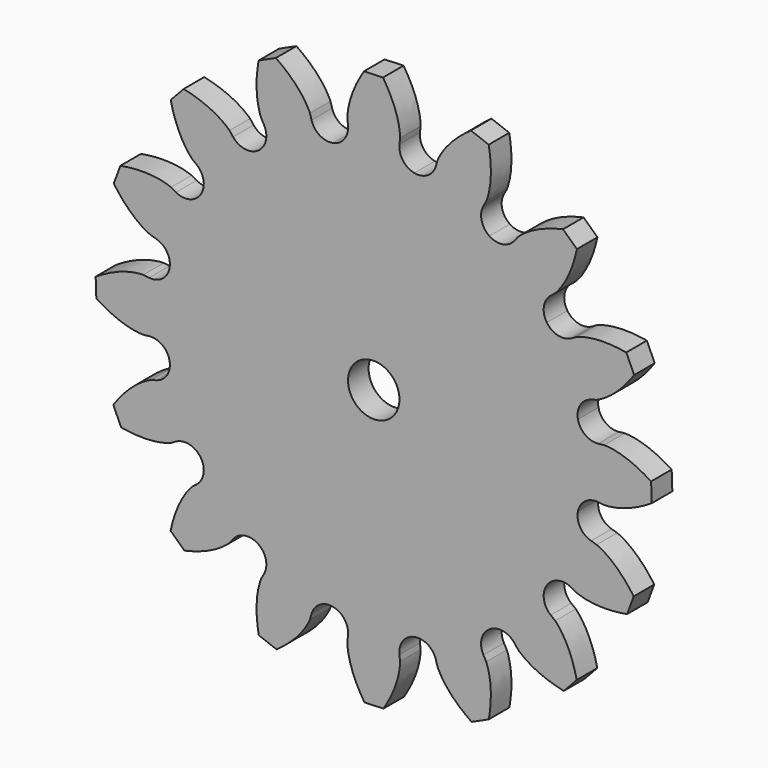
from build123d import *

# Parameters (mm, degrees)
F1_R     = 20.25
F2_DEPTH = 2.5
F4_DEPTH = 2.5
F5_COUNT = 16
F6_R     = 2.5
F7_DEPTH = 2.5010001


with BuildPart() as f2:
    # F1 (on Front) → F2 (new body)
    with BuildSketch(Plane.XZ):
        Circle(F1_R)
    extrude(amount=F2_DEPTH)

    # F3 (on Front) → F4 (join)
    with BuildSketch(Plane.XZ):
        with BuildLine():
            Line((2.501493717, 21.8474319576), (2.5654751255, 22.4062298703))
            add(Edge.make_bspline(
                [(2.5654751255, 22.4062298703), (2.5722302046, 22.5041299531), (2.5280812859, 23.392024488), (2.0217706958, 25.1203618373), (1.2383732447, 26.5188041263), (0.9036927257, 27.048160041)],
                knots=[0, 0, 0, 0, 0.0943076993, 0.2574918928, 0.3558520384, 0.3558520384, 0.3558520384, 0.3558520384], degree=3))
            Line((0.9036927257, 27.048160041), (-0.9443977609, 26.9834785168))
            add(Edge.make_bspline(
                [(-2.5654751255, 22.4062298703), (-2.5722302046, 22.5041299531), (-2.5280812859, 23.392024488), (-2.0274723322, 25.1008987818), (-1.2622826417, 26.4759812142), (-0.9443977609, 26.9834785168)],
                knots=[0, 0, 0, 0, 0.0943076993, 0.2574918928, 0.3518447374, 0.3518447374, 0.3518447374, 0.3518447374], degree=3))
            Line((-2.5654751255, 22.4062298703), (-2.501493717, 21.8474319576))
            ThreePointArc((-2.501493717, 21.8474319576), (-2.8383699375, 20.5713815229), (-3.9505790208, 19.8609019282))
            Line((-3.9505790208, 19.8609019282), (0, 0))
            Line((0, 0), (3.9505790208, 19.8609019282))
            ThreePointArc((3.9505790208, 19.8609019282), (2.8383699375, 20.5713815229), (2.501493717, 21.8474319576))
        make_face()
    extrude(amount=F4_DEPTH)

    # F5: F2 ×16 about axis
    f5_axis = Axis((0, 0, 0), (0, -1, 0))


with BuildPart() as f2_1:
    add(f2.part)
    for i in range(1, F5_COUNT):
        add(f2.part.rotate(f5_axis, i * 360 / F5_COUNT))

    # F6 (on face) → F7 (cut, through all)
    with BuildSketch(Plane.XZ.offset(2.5)):
        Circle(F6_R)
    extrude(amount=-F7_DEPTH, mode=Mode.SUBTRACT)


solid = f2_1.part
